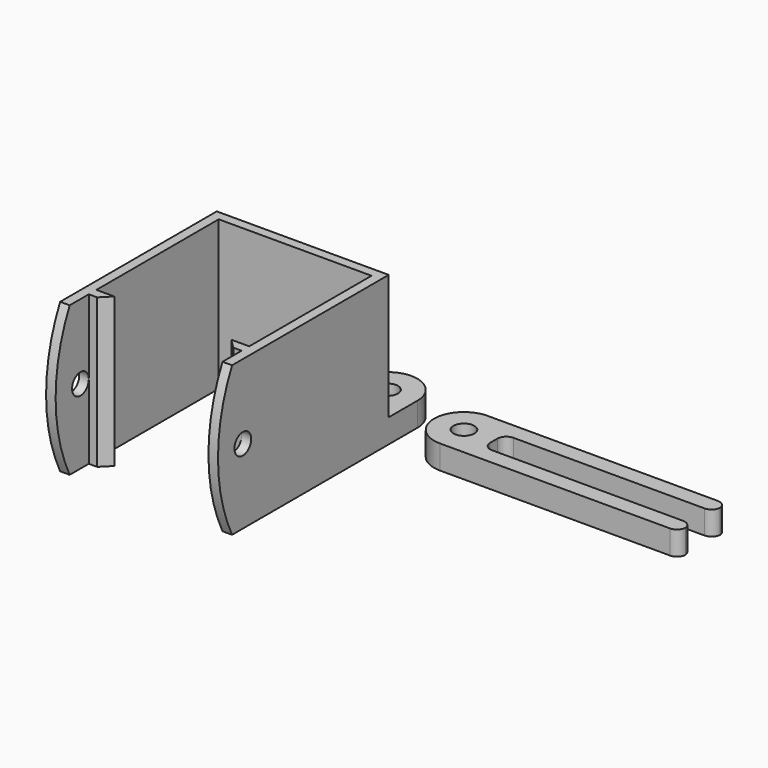
from build123d import *

# Parameters (mm, degrees)
F1_DEPTH     = 25
F2_SIZE      = 1.59999
F4_DEPTH     = 1.6
F6_DEPTH     = 1.6
F7_R         = 1.75
F8_DEPTH     = 50
F10_DEPTH    = 4
F11_R        = 1.75
F12_DEPTH    = 25.001
F13_W        = 45
F13_H        = 10
F14_DEPTH    = 4
F15_R        = 4.99999
F16_R        = 1.75
F17_DEPTH    = 4.001
F18_W        = 35
F18_H        = 4.5
F19_DEPTH    = 4.001
F20_T1_DEPTH = 4
F20_T3_DEPTH = 11.5


# Not quite as in the source:
# - a fillet or chamfer that OpenCascade refuses, or shapes differently, is made with other operations: its cross-section is extruded or revolved along the edge and cut away or added
# - a fillet or chamfer is up to 0.001 mm smaller than in the source, because OpenCascade refuses the exact size


with BuildPart() as f1:
    # F0 (on Top) → F1 (new body)
    with BuildSketch(Plane.XY):
        Polygon((-25.6, 0), (0, 0), (0, -25.6), (-3, -25.6), (-3, -27.2), (0, -27.2), (0, -31.2), (1.6, -31.2), (1.6, 1.6), (-27.2, 1.6), (-27.2, -31.2), (-25.6, -31.2), (-25.6, -27.2), (-22.6, -27.2), (-22.6, -25.6), (-25.6, -25.6), align=None)
    extrude(amount=F1_DEPTH)

    # F2 (size 1.6 in the source; OpenCascade refuses exactly that, so slightly less here)
    f2_edges = [f1.edges().sort_by_distance(p)[0] for p in [
        (-22.6, -27.2, 12.5),
        (-3, -27.2, 12.5),
    ]]
    chamfer(f2_edges, length=F2_SIZE)

    # F3 (on face) → F4 (join, through all)
    with BuildSketch(Plane(origin=(-27.2, 0, 0), x_dir=(0, -1, 0), z_dir=(-1, 0, 0))):
        with BuildLine():
            Line((31.2, 25), (31.2, 0))
            ThreePointArc((31.2, 0), (34.1450603673, 12.5), (31.2, 25))
        make_face()
    extrude(amount=-F4_DEPTH)

    # F5 (on face) → F6 (join, through all)
    with BuildSketch(Plane.YZ.offset(1.6)):
        with BuildLine():
            Line((-31.2, 0), (-31.2, 25))
            ThreePointArc((-31.2, 25), (-34.1450603673, 12.5), (-31.2, 0))
        make_face()
    extrude(amount=-F6_DEPTH)

    # F7 (on face) → F8 (cut, symmetric)
    with BuildSketch(Plane.YZ.offset(-25.6)):
        with Locations((-28.95, 12.5)):
            Circle(F7_R)
    extrude(amount=F8_DEPTH, both=True, mode=Mode.SUBTRACT)

    # F9 (on Top) → F10 (join)
    with BuildSketch(Plane.XY):
        with BuildLine():
            ThreePointArc((-8.4, 7.6), (-3.4, 2.6), (1.6, 7.6))
            ThreePointArc((1.6, 7.6), (-3.4, 12.6), (-8.4, 7.6))
        make_face()
        with BuildLine():
            Line((1.6, 1.6), (1.6, 7.6))
            ThreePointArc((1.6, 7.6), (-3.4, 2.6), (-8.4, 7.6))
            Line((-8.4, 7.6), (-8.4, 1.6))
            Line((-8.4, 1.6), (1.6, 1.6))
        make_face()
    extrude(amount=F10_DEPTH)

    # F11 (on Top) → F12 (cut, through all)
    with BuildSketch(Plane.XY):
        with Locations((-3.4, 7.6)):
            Circle(F11_R)
    extrude(amount=F12_DEPTH, mode=Mode.SUBTRACT)


with BuildPart() as f14:
    # F13 (on Top) → F14 (new body)
    with BuildSketch(Plane.XY):
        with Locations((28.9799958316, 5)):
            Rectangle(F13_W, F13_H)
    extrude(amount=F14_DEPTH)

    # F15 (radius 5 in the source; OpenCascade refuses exactly that, so slightly less here)
    f15_edges = [f14.edges().sort_by_distance(p)[0] for p in [
        (6.479996, 0, 2),
        (6.479996, 10, 2),
    ]]
    fillet(f15_edges, radius=F15_R)

    # F16 (on face) → F17 (cut, through all)
    with BuildSketch(Plane.XY.offset(4)):
        with Locations((11.4799958316, 5)):
            Circle(F16_R)
    extrude(amount=-F17_DEPTH, mode=Mode.SUBTRACT)

    # F18 (on face) → F19 (cut, through all)
    with BuildSketch(Plane.XY.offset(4)):
        with Locations((33.9799958316, 5)):
            Rectangle(F18_W, F18_H)
    extrude(amount=-F19_DEPTH, mode=Mode.SUBTRACT)

    # F20: fillet of radius 1.5 on 6 edges, made by hand

    # F20_s2 → F20_t1 (join)
    with BuildSketch(Plane.XY):
        with BuildLine():
            ThreePointArc((17.9799958316, 7.25), (16.9193356598, 6.8106601718), (16.4799958316, 5.75))
            Line((16.4799958316, 5.75), (16.4799958316, 7.25))
            Line((16.4799958316, 7.25), (17.9799958316, 7.25))
        make_face()
        with BuildLine():
            ThreePointArc((16.4799958316, 4.25), (16.9193356598, 3.1893398282), (17.9799958316, 2.75))
            Line((17.9799958316, 2.75), (16.4799958316, 2.75))
            Line((16.4799958316, 2.75), (16.4799958316, 4.25))
        make_face()
    extrude(amount=F20_T1_DEPTH)

    # F20_s4 → F20_t3 (cut)
    with BuildSketch(Plane.XY.offset(-3.75)):
        with BuildLine():
            ThreePointArc((51.4799958316, 8.75), (51.0406560034, 7.6893398282), (49.9799958316, 7.25))
            Line((49.9799958316, 7.25), (51.4799958316, 7.25))
            Line((51.4799958316, 7.25), (51.4799958316, 8.75))
        make_face()
        with BuildLine():
            ThreePointArc((49.9799958316, 10), (51.0406560034, 9.5606601718), (51.4799958316, 8.5))
            Line((51.4799958316, 8.5), (51.4799958316, 10))
            Line((51.4799958316, 10), (49.9799958316, 10))
        make_face()
        with BuildLine():
            ThreePointArc((51.4799958316, 1.25), (51.0406560034, 2.3106601718), (49.9799958316, 2.75))
            Line((49.9799958316, 2.75), (51.4799958316, 2.75))
            Line((51.4799958316, 2.75), (51.4799958316, 1.25))
        make_face()
        with BuildLine():
            ThreePointArc((49.9799958316, 0), (51.0406560034, 0.4393398282), (51.4799958316, 1.5))
            Line((51.4799958316, 1.5), (51.4799958316, 0))
            Line((51.4799958316, 0), (49.9799958316, 0))
        make_face()
    extrude(amount=F20_T3_DEPTH, mode=Mode.SUBTRACT)


solid = Compound([f1.part, f14.part])
